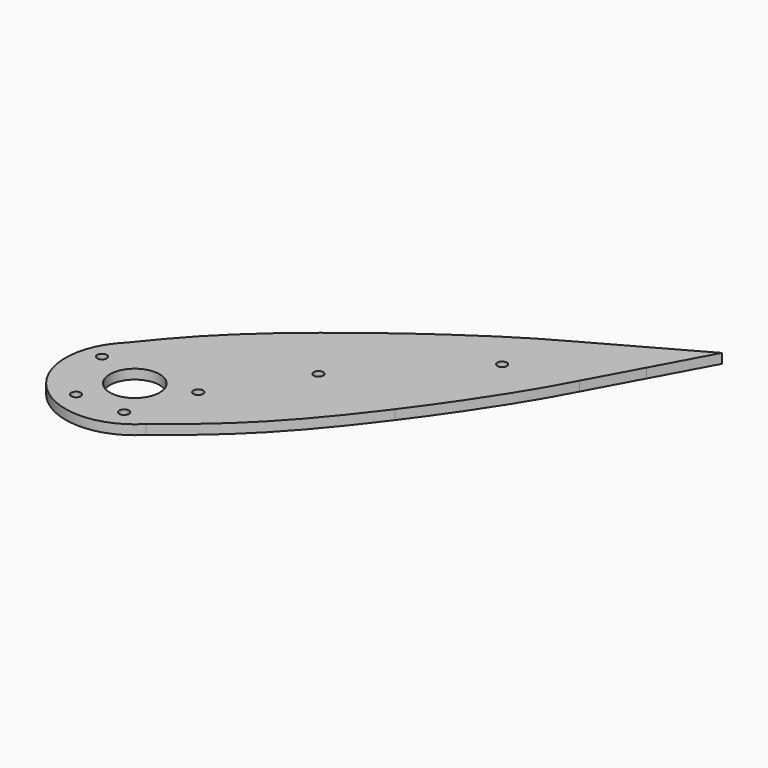
from build123d import *

# Parameters (mm, degrees)
F0_R     = 1.5875
F1_DEPTH = 3.175


with BuildPart() as f1:
    # F0 (on Top) → F1 (new body)
    with BuildSketch(Plane.XY):
        with BuildLine():
            ThreePointArc((48.298852367, 25.3648877175), (46.5534190331, 34.1258622353), (41.5836577474, 41.5489805011))
            ThreePointArc((41.5836577474, 41.5489805011), (25.5683959748, 48.2245206641), (9.478505781, 41.7309176838))
            ThreePointArc((9.478505781, 41.7309176838), (9.2940469865, 9.1807949339), (41.8436252726, 9.4443655555))
            ThreePointArc((41.8436252726, 9.4443655555), (46.6236666053, 16.7751702782), (48.298852367, 25.3648877175))
        make_face()
        with BuildLine():
            ThreePointArc((19.088852367, 11.0773877175), (16.3788203518, 9.9548557024), (17.501352367, 12.6648877175))
            ThreePointArc((17.501352367, 12.6648877175), (18.6238843821, 12.1999197327), (19.088852367, 11.0773877175))
        make_face(mode=Mode.SUBTRACT)
        with Locations((9.525, 31.75)):
            Circle(F0_R, mode=Mode.SUBTRACT)
        with BuildLine():
            Line((38.1080227106, 38.0648877175), (38.138852367, 38.0648877175))
            Line((38.138852367, 38.0648877175), (38.138852367, 12.6648877175))
            Line((38.138852367, 12.6648877175), (33.669537083, 12.6648877175))
            ThreePointArc((33.669537083, 12.6648877175), (34.5718551189, 12.110760332), (34.925, 11.1125))
            ThreePointArc((34.925, 11.1125), (32.339239668, 9.8781448811), (33.005462917, 12.6648877175))
            Line((33.005462917, 12.6648877175), (17.501352367, 12.6648877175))
            Line((17.501352367, 12.6648877175), (12.738852367, 12.6648877175))
            Line((12.738852367, 12.6648877175), (12.738852367, 38.0648877175))
            Line((12.738852367, 38.0648877175), (38.1080227106, 38.0648877175))
        make_face(mode=Mode.SUBTRACT)
        with Locations((41.275, 31.75)):
            Circle(F0_R, mode=Mode.SUBTRACT)
        with BuildLine():
            Line((57.9526965359, 57.9578523511), (41.5836577474, 41.5489805011))
            ThreePointArc((41.5836577474, 41.5489805011), (46.5534190331, 34.1258622353), (48.298852367, 25.3648877175))
            ThreePointArc((48.298852367, 25.3648877175), (46.6236666053, 16.7751702782), (41.8436252726, 9.4443655555))
            add(Edge.make_bspline(
                [(86.8310062503, 56.0153192292), (83.249706502, 51.2144143314), (63.5484661138, 26.0258843806), (51.3080659428, 17.112891847), (41.8436252726, 9.4443655555)],
                knots=[0.7406020956, 0.7406020956, 0.7406020956, 0.7406020956, 0.7871603002, 1, 1, 1, 1], degree=3))
            ThreePointArc((86.8310062503, 56.0153192292), (75.7950461349, 59.6100245839), (66.4012027896, 66.4269175316))
            Line((66.4012027896, 66.4269175316), (60.1950306165, 60.2056430155))
            ThreePointArc((60.1950306165, 60.2056430155), (60.540152928, 59.6901486915), (60.6613635762, 59.0817476833))
            ThreePointArc((60.6613635762, 59.0817476833), (59.6822645844, 57.6154583315), (57.9526965359, 57.9578523511))
        make_face()
        with BuildLine():
            ThreePointArc((9.478505781, 41.7309176838), (25.5683959748, 48.2245206641), (41.5836577474, 41.5489805011))
            Line((41.5836577474, 41.5489805011), (57.9526965359, 57.9578523511))
            ThreePointArc((57.9526965359, 57.9578523511), (57.949968244, 60.2029147236), (60.1950306165, 60.2056430155))
            Line((60.1950306165, 60.2056430155), (66.4012027896, 66.4269175316))
            ThreePointArc((66.4012027896, 66.4269175316), (59.7830008839, 75.3788925735), (56.1057766209, 85.88681698))
            add(Edge.make_bspline(
                [(9.478505781, 41.7309176838), (17.0929440337, 51.1603431722), (26.371548526, 62.5901940603), (51.3329129213, 82.2718852167), (56.1057766209, 85.88681698)],
                knots=[0, 0, 0, 0, 0.211634739, 0.2581952867, 0.2581952867, 0.2581952867, 0.2581952867], degree=3))
        make_face()
        with BuildLine():
            Line((89.1799820166, 89.261127534), (66.4012027896, 66.4269175316))
            ThreePointArc((66.4012027896, 66.4269175316), (75.7950461349, 59.6100245839), (86.8310062503, 56.0153192292))
            add(Edge.make_bspline(
                [(113.9930376147, 98.1438093202), (107.5652173309, 85.5841385514), (97.0153094729, 69.6678684875), (86.8310062503, 56.0153192292)],
                knots=[0.6082024344, 0.6082024344, 0.6082024344, 0.6082024344, 0.7406020956, 0.7406020956, 0.7406020956, 0.7406020956], degree=3))
            Line((113.9930376147, 98.1438093202), (105.9976837923, 106.1197541654))
            Line((105.9976837923, 106.1197541654), (96.2377675544, 96.3360877642))
            ThreePointArc((96.2377675544, 96.3360877642), (97.3240460353, 94.7135604092), (97.7055586597, 92.7986076491))
            ThreePointArc((97.7055586597, 92.7986076491), (94.6238275456, 88.1834363993), (89.1799820166, 89.261127534))
        make_face()
        with BuildLine():
            add(Edge.make_bspline(
                [(56.1057766209, 85.88681698), (69.7989441385, 96.2579210625), (85.7273267139, 107.1699447817), (98.2606169463, 113.8380390341)],
                knots=[0.2581952867, 0.2581952867, 0.2581952867, 0.2581952867, 0.3917757571, 0.3917757571, 0.3917757571, 0.3917757571], degree=3))
            ThreePointArc((56.1057766209, 85.88681698), (59.7830008839, 75.3788925735), (66.4012027896, 66.4269175316))
            Line((66.4012027896, 66.4269175316), (89.1799820166, 89.261127534))
            ThreePointArc((89.1799820166, 89.261127534), (89.1713946704, 96.327500418), (96.2377675544, 96.3360877642))
            Line((96.2377675544, 96.3360877642), (105.9976837923, 106.1197541654))
            Line((105.9976837923, 106.1197541654), (98.2606169463, 113.8380390341))
        make_face()
        with BuildLine():
            Line((38.138852367, 12.6648877175), (38.138852367, 38.0648877175))
            Line((38.138852367, 38.0648877175), (38.1080227106, 38.0648877175))
            Line((38.1080227106, 38.0648877175), (12.738852367, 38.0648877175))
            Line((12.738852367, 38.0648877175), (12.738852367, 12.6648877175))
            Line((12.738852367, 12.6648877175), (17.501352367, 12.6648877175))
            Line((17.501352367, 12.6648877175), (33.005462917, 12.6648877175))
            ThreePointArc((33.005462917, 12.6648877175), (33.3375, 12.7), (33.669537083, 12.6648877175))
            Line((33.669537083, 12.6648877175), (38.138852367, 12.6648877175))
        make_face()
        with BuildLine():
            ThreePointArc((33.6445749551, 25.3648877175), (17.8596626631, 22.2200877834), (31.2341189545, 31.1742567343))
            ThreePointArc((31.2341189545, 31.1742567343), (33.0180420708, 28.5096876517), (33.6445749551, 25.3648877175))
        make_face(mode=Mode.SUBTRACT)
        with BuildLine():
            Line((105.9976837923, 106.1197541654), (113.9930376147, 98.1438093202))
            add(Edge.make_bspline(
                [(119.0607801069, 119.1260976819), (121.7354589285, 116.3963605732), (119.2349256659, 108.3862220235), (113.9930376147, 98.1438093202)],
                knots=[0.5002304981, 0.5002304981, 0.5002304981, 0.5002304981, 0.6082024344, 0.6082024344, 0.6082024344, 0.6082024344], degree=3))
            ThreePointArc((119.0607801069, 119.1260976819), (119.038672719, 119.1482070061), (119.0165467814, 119.1702977666))
            Line((119.0165467814, 119.1702977666), (105.9976837923, 106.1197541654))
        make_face()
        with BuildLine():
            add(Edge.make_bspline(
                [(98.2606169463, 113.8380390341), (108.3812043908, 119.2225015111), (116.2880200857, 121.8397075452), (119.0165467814, 119.1702977666)],
                knots=[0.3917757571, 0.3917757571, 0.3917757571, 0.3917757571, 0.4996415136, 0.4996415136, 0.4996415136, 0.4996415136], degree=3))
            Line((98.2606169463, 113.8380390341), (105.9976837923, 106.1197541654))
            Line((105.9976837923, 106.1197541654), (119.0165467814, 119.1702977666))
        make_face()
        with BuildLine():
            Line((132.9733085625, 133.1610224797), (119.0165467814, 119.1702977666))
            add(Edge.make_bspline(
                [(119.0165467814, 119.1702977666), (119.0314454842, 119.1557218627), (119.0461897944, 119.1409883361), (119.0607801069, 119.1260976819)],
                knots=[0.4996415136, 0.4996415136, 0.4996415136, 0.4996415136, 0.5002304981, 0.5002304981, 0.5002304981, 0.5002304981], degree=3))
            ThreePointArc((119.0607801069, 119.1260976819), (121.0771249041, 116.9399007111), (122.9126341528, 114.5998132483))
            Line((122.9126341528, 114.5998132483), (132.9733085625, 133.1610224797))
        make_face()
        with BuildLine():
            Line((132.9733085625, 133.1610224797), (114.6029810942, 122.9350930852))
            ThreePointArc((114.6029810942, 122.9350930852), (116.8831644106, 121.1387446745), (119.0165467814, 119.1702977666))
            Line((119.0165467814, 119.1702977666), (132.9733085625, 133.1610224797))
        make_face()
        with BuildLine():
            ThreePointArc((96.2377675544, 96.3360877642), (89.1713946704, 96.327500418), (89.1799820166, 89.261127534))
            Line((89.1799820166, 89.261127534), (91.5877077452, 91.6747123169))
            ThreePointArc((91.5877077452, 91.6747123169), (91.5849794533, 93.9197746894), (93.8300418258, 93.9225029813))
            Line((93.8300418258, 93.9225029813), (96.2377675544, 96.3360877642))
        make_face()
        with BuildLine():
            Line((91.5877077452, 91.6747123169), (89.1799820166, 89.261127534))
            ThreePointArc((89.1799820166, 89.261127534), (94.6238275456, 88.1834363993), (97.7055586597, 92.7986076491))
            ThreePointArc((97.7055586597, 92.7986076491), (97.3240460353, 94.7135604092), (96.2377675544, 96.3360877642))
            Line((96.2377675544, 96.3360877642), (93.8300418258, 93.9225029813))
            ThreePointArc((93.8300418258, 93.9225029813), (94.1751641373, 93.4070086573), (94.2963747855, 92.7986076491))
            ThreePointArc((94.2963747855, 92.7986076491), (93.3172757937, 91.3323182973), (91.5877077452, 91.6747123169))
        make_face()
        with BuildLine():
            add(Edge.make_bspline(
                [(119.0607801069, 119.1260976819), (121.7354589285, 116.3963605732), (119.2349256659, 108.3862220235), (113.9930376147, 98.1438093202)],
                knots=[0.5002304981, 0.5002304981, 0.5002304981, 0.5002304981, 0.6082024344, 0.6082024344, 0.6082024344, 0.6082024344], degree=3))
            Line((113.9930376147, 98.1438093202), (122.9126341528, 114.5998132483))
            ThreePointArc((122.9126341528, 114.5998132483), (121.0771249041, 116.9399007111), (119.0607801069, 119.1260976819))
        make_face()
        with BuildLine():
            ThreePointArc((119.0165467814, 119.1702977666), (116.8831644106, 121.1387446745), (114.6029810942, 122.9350930852))
            Line((114.6029810942, 122.9350930852), (98.2606169463, 113.8380390341))
            add(Edge.make_bspline(
                [(98.2606169463, 113.8380390341), (108.3812043908, 119.2225015111), (116.2880200857, 121.8397075452), (119.0165467814, 119.1702977666)],
                knots=[0.3917757571, 0.3917757571, 0.3917757571, 0.3917757571, 0.4996415136, 0.4996415136, 0.4996415136, 0.4996415136], degree=3))
        make_face()
        with BuildLine():
            add(Edge.make_bspline(
                [(119.0165467814, 119.1702977666), (119.0314454842, 119.1557218627), (119.0461897944, 119.1409883361), (119.0607801069, 119.1260976819)],
                knots=[0.4996415136, 0.4996415136, 0.4996415136, 0.4996415136, 0.5002304981, 0.5002304981, 0.5002304981, 0.5002304981], degree=3))
            ThreePointArc((119.0165467814, 119.1702977666), (119.038672719, 119.1482070061), (119.0607801069, 119.1260976819))
        make_face()
    extrude(amount=F1_DEPTH)


solid = f1.part
